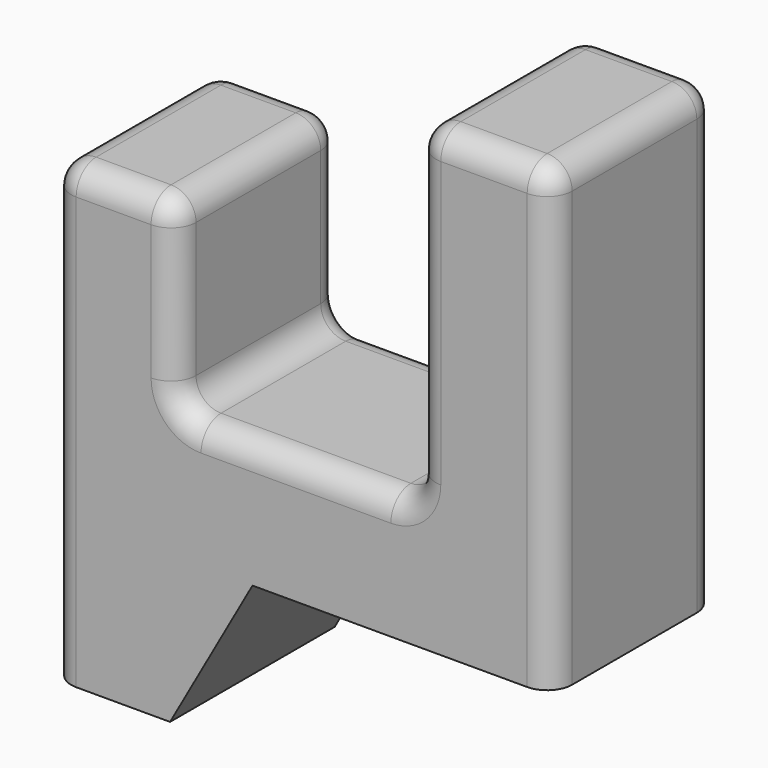
from build123d import *

# Parameters (mm, degrees)
F1_DEPTH = 20.6
F2_R     = 5


with BuildPart() as f1:
    # F0 (on Front) → F1 (new body, symmetric)
    with BuildSketch(Plane.XZ):
        Polygon((-82.7489259505, 37), (-107.7489259505, 37), (-107.7489259505, -54.4), (-83.9489259505, -54.4), (-67.4489259505, -25), (-7.4489259505, -25), (-7.4489259505, 67), (-34.7489259505, 67), (-34.7489259505, 0), (-82.7489259505, 0), align=None)
    extrude(amount=F1_DEPTH, both=True)

    # F2
    f2_edges = [f1.edges().sort_by_distance(p)[0] for p in [
        (-107.748926, 0, 37),
        (-82.748926, 0, 37),
        (-95.248926, -20.6, 37),
        (-95.248926, 20.6, 37),
        (-82.748926, -20.6, 18.5),
        (-82.748926, 0, 0),
        (-82.748926, 20.6, 18.5),
        (-58.748926, 20.6, 0),
        (-58.748926, -20.6, 0),
        (-34.748926, 0, 0),
        (-34.748926, 0, 67),
        (-21.098926, -20.6, 67),
        (-21.098926, 20.6, 67),
        (-7.448926, 0, 67),
        (-34.748926, -20.6, 33.5),
        (-7.448926, -20.6, 21),
        (-7.448926, 20.6, 21),
        (-107.748926, -20.6, -8.7),
        (-107.748926, 20.6, -8.7),
        (-34.748926, 20.6, 33.5),
    ]]
    fillet(f2_edges, radius=F2_R)


solid = f1.part
